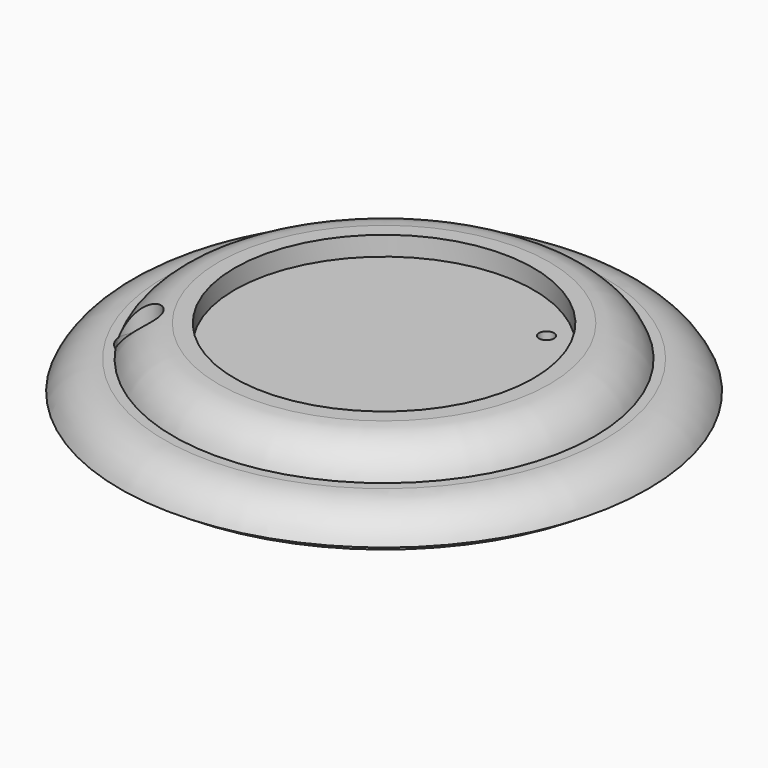
from build123d import *

# Parameters (mm, degrees)
F0_R      = 27.8603665739
F1_DEPTH  = 3.048
F4_R      = 26.2786257822
F5_DEPTH  = 1.016
F6_R      = 22.2176168744
F7_DEPTH  = 3.302
F9_R      = 15.773437446
F10_DEPTH = 2.032
F11_R     = 2.2956006308
F12_DEPTH = 21.336
F13_R     = 2.0464830212
F14_DEPTH = 25.4
F15_R     = 0.7900286513
F16_DEPTH = 25.4


# Not quite as in the source:
# - a fillet or chamfer that OpenCascade refuses, or shapes differently, is made with other operations: its cross-section is extruded or revolved along the edge and cut away or added


with BuildPart() as f1:
    # F0 (on Top) → F1 (new body)
    with BuildSketch(Plane.XY):
        Circle(F0_R)
    extrude(amount=F1_DEPTH)

    # F2: fillet of radius 5.08 on 1 edges, made by hand

    # F2_s1 → F2_t2 (revolve, cut)
    with BuildSketch(Plane.XZ):
        with BuildLine():
            ThreePointArc((27.8603665739, 0), (25.9869002599, 2.2182329348), (23.2044696678, 3.048))
            Line((23.2044696678, 3.048), (27.8603665739, 3.048))
            Line((27.8603665739, 3.048), (27.8603665739, 0))
        make_face()
    revolve(axis=Axis((0, 0, 3.048), (0, 0, 1)), mode=Mode.SUBTRACT)

    # F4 (on face) → F5 (join)
    with BuildSketch(Plane(origin=(0, 0, 0), x_dir=(1, 0, 0), z_dir=(0, 0, -1))):
        Circle(F4_R)
    extrude(amount=F5_DEPTH)

    # F6 (on face) → F7 (join)
    with BuildSketch(Plane.XY.offset(3.048)):
        Circle(F6_R)
    extrude(amount=F7_DEPTH)

    # F8: fillet of radius 5.08 on 1 edges, made by hand

    # F8_s1 → F8_t2 (revolve, cut)
    with BuildSketch(Plane.XZ):
        with BuildLine():
            ThreePointArc((22.2176168744, 3.048), (20.3549739793, 5.4436458882), (17.4589283996, 6.35))
            Line((17.4589283996, 6.35), (22.2176168744, 6.35))
            Line((22.2176168744, 6.35), (22.2176168744, 3.048))
        make_face()
    revolve(axis=Axis((0, 0, 6.35), (0, 0, 1)), mode=Mode.SUBTRACT)

    # F9 (on face) → F10 (cut)
    with BuildSketch(Plane.XY.offset(6.35)):
        Circle(F9_R)
    extrude(amount=-F10_DEPTH, mode=Mode.SUBTRACT)

    # F11 (on face) → F12 (cut)
    with BuildSketch(Plane.XY.offset(3.048)):
        with Locations((-17.1565320343, -10.5084851384)):
            Circle(F11_R)
    extrude(amount=-F12_DEPTH, mode=Mode.SUBTRACT)

    # F13 (on face) → F14 (cut)
    with BuildSketch(Plane.XY.offset(6.35)):
        with Locations((-17.3885338008, -10.6187639758)):
            Circle(F13_R)
    extrude(amount=-F14_DEPTH, mode=Mode.SUBTRACT)

    # F15 (on face) → F16 (cut)
    with BuildSketch(Plane.XY.offset(4.318)):
        with Locations((9.4199227169, 9.6543869004)):
            Circle(F15_R)
    extrude(amount=-F16_DEPTH, mode=Mode.SUBTRACT)


solid = f1.part
